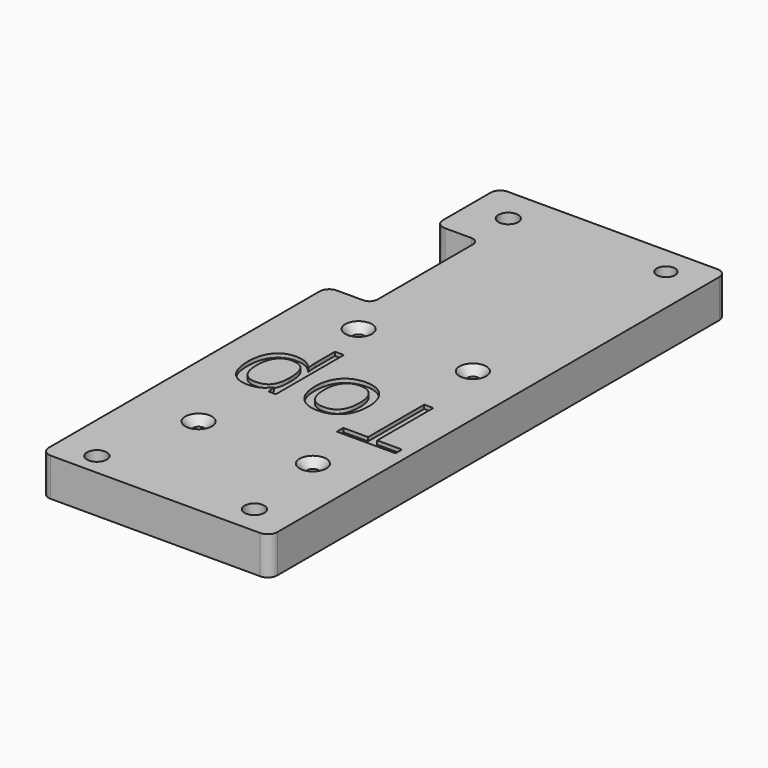
from build123d import *

# Parameters (mm, degrees)
F0_R         = 3.0504144311
F0_R_2       = 1.905
F0_R_3       = 3.302
F1_DEPTH     = 12.7
F2_R         = 3.175
F3_SIZE      = 2.54
F4_TEXT_SIZE = 36.5489679906
F5_DEPTH     = 1.27
F6_ANGLE     = 180
F7_ANGLE     = 180
F10_DEPTH    = 39.878


# Not quite as in the source:
# - Text() gives the source's letters only with a copy of the font that has no kerning and outlines rounded to 1/6400 em; it was checked with that copy


with BuildPart() as f1:
    # F0 (on Top) → F1 (new body)
    with BuildSketch(Plane.XY):
        with BuildLine():
            Line((-35.9423857893, -103.7576142107), (40.2576142107, -103.7576142107))
            Line((40.2576142107, -103.7576142107), (40.2576142107, -77.4861343209))
            Line((40.2576142107, -77.4861343209), (28.1930232728, -77.4861343209))
            ThreePointArc((28.1930232728, -77.4861343209), (26.3969720485, -76.7421855451), (25.6530232728, -74.9461343209))
            Line((25.6530232728, -74.9461343209), (25.6530232728, -35.0238956982))
            ThreePointArc((25.6530232728, -35.0238956982), (26.3969720485, -33.227844474), (28.1930232728, -32.4838956982))
            Line((28.1930232728, -32.4838956982), (40.2576142107, -32.4838956982))
            Line((40.2576142107, -32.4838956982), (40.2576142107, 86.7423857893))
            Line((40.2576142107, 86.7423857893), (-35.9423857893, 86.7423857893))
            Line((-35.9423857893, 86.7423857893), (-35.9423857893, -103.7576142107))
        make_face()
        with Locations((-23.2423857893, -94.2326142107)):
            Circle(F0_R, mode=Mode.SUBTRACT)
        with Locations((-19.05, -19.05)):
            Circle(F0_R_2, mode=Mode.SUBTRACT)
        with Locations((27.5576142107, -92.075)):
            Circle(F0_R_3, mode=Mode.SUBTRACT)
        with Locations((19.05, -19.05)):
            Circle(F0_R_2, mode=Mode.SUBTRACT)
        with Locations((-19.05, 47.625)):
            Circle(F0_R_2, mode=Mode.SUBTRACT)
        with Locations((-23.2423857893, 77.2173857893)):
            Circle(F0_R_3, mode=Mode.SUBTRACT)
        with Locations((19.05, 47.625)):
            Circle(F0_R_2, mode=Mode.SUBTRACT)
        with Locations((27.5576142107, 79.375)):
            Circle(F0_R_3, mode=Mode.SUBTRACT)
    extrude(amount=F1_DEPTH)

    # F2
    f2_edges = [f1.edges().sort_by_distance(p)[0] for p in [
        (-35.942386, -103.757614, 6.35),
        (40.257614, -103.757614, 6.35),
        (40.257614, 86.742386, 6.35),
        (-35.942386, 86.742386, 6.35),
        (40.257614, -32.483896, 6.35),
        (40.257614, -77.486134, 6.35),
    ]]
    fillet(f2_edges, radius=F2_R)

    # F3
    f3_edges = [f1.edges().sort_by_distance(p)[0] for p in [
        (17.145, -19.05, 12.7),
        (-20.955, -19.05, 12.7),
        (-20.955, 47.625, 12.7),
        (17.145, 47.625, 12.7),
        (24.255614, 79.375, 0),
        (-26.544386, 77.217386, 0),
        (24.255614, -92.075, 0),
        (-26.2928, -94.232614, 0),
    ]]
    chamfer(f3_edges, length=F3_SIZE)

    # F4 (on face) → F5 (cut)
    with BuildSketch(Plane.XY.offset(12.7)):
        with Locations((-32.5171613852, 3.5560044926)):
            Text('Top', F4_TEXT_SIZE, font='Open Sans', text_align=(TextAlign.LEFT, TextAlign.BOTTOM))
    extrude(amount=-F5_DEPTH, mode=Mode.SUBTRACT)


with BuildPart() as f1_1:
    # F6: moved
    add(f1.part.rotate(Axis((-35.9423857893, -8.5076142107, 12.7), (0, 1, 0)), F6_ANGLE))


with BuildPart() as f1_2:
    # F7: moved
    add(f1_1.part.rotate(Axis((-74.0423857893, -103.7576142107, 25.4), (1, 0, 0)), F7_ANGLE))

    # F9 (on offset) → F10 (cut)
    with BuildSketch(Plane(origin=(0, -132.7136142107, 0), x_dir=(-1, 0, 0), z_dir=(0, 1, 0))):
        Polygon((98.3419641852, 23.7634535879), (98.3419641852, 39.7620732109), (90.2660042047, 23.7634535879), align=None)
    extrude(amount=-F10_DEPTH, mode=Mode.SUBTRACT)


with BuildPart() as f1_3:
    # F11: moved
    add(f1_2.part.moved(Location((71.12, 190.5, 0))))


solid = f1_3.part
